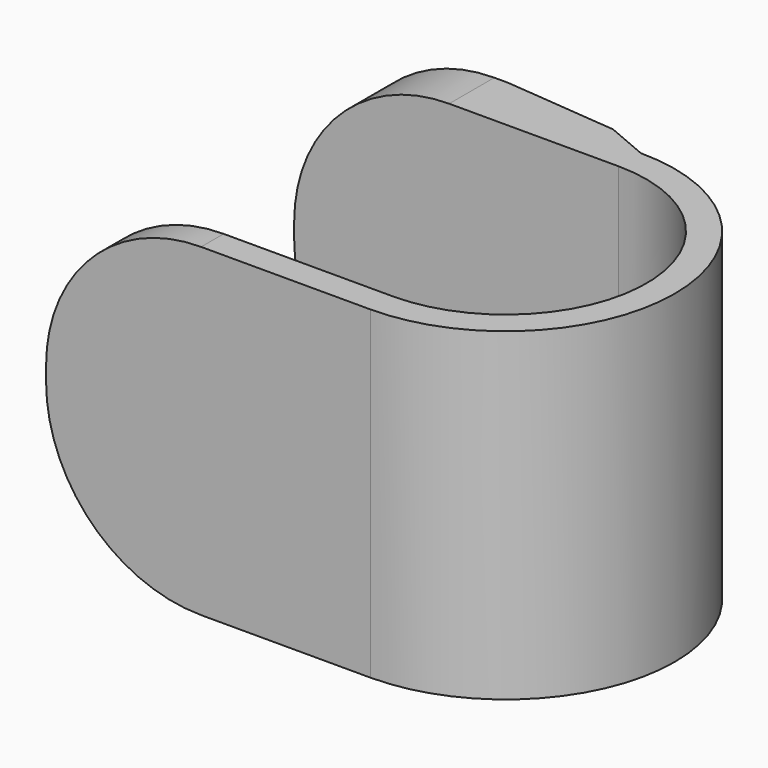
from build123d import *

# Parameters (mm, degrees)
F0_W           = 23
F0_H           = 2
F1_DEPTH       = 23
F3_D           = 1
F3_DEPTH       = 3
F3_CBORE_D     = 19.5
F3_CBORE_DEPTH = 3
F3_TIP         = 0.3004303095
F4_R           = 11
F5_T1_DEPTH    = 80.1913118923
F6_T4_DEPTH    = 38.5721694425
F6_S5_R        = 12
F6_T6_DEPTH    = 21


# Not quite as in the source:
# - a fillet or chamfer that OpenCascade refuses, or shapes differently, is made with other operations: its cross-section is extruded or revolved along the edge and cut away or added


with BuildPart() as f1:
    # F0 (on Top) → F1 (new body)
    with BuildSketch(Plane.XY):
        with BuildLine():
            Line((-8.3816226795, 2), (-8.3816226795, 0))
            Line((-8.3816226795, 0), (14.6183773205, 0))
            ThreePointArc((14.6183773205, 0), (24.6183773205, -10), (14.6183773205, -20))
            Line((14.6183773205, -20), (-8.3816226795, -20))
            Line((-8.3816226795, -20), (-8.3816226795, -22))
            Line((-8.3816226795, -22), (14.6183773205, -22))
            ThreePointArc((14.6183773205, -22), (26.6183773205, -10), (14.6183773205, 2))
            Line((14.6183773205, 2), (-8.3816226795, 2))
        make_face()
        with Locations((3.1183773205, 3)):
            Rectangle(F0_W, F0_H)
    extrude(amount=F1_DEPTH)

    # F3
    with Locations(Plane(origin=(0, 4, 0), x_dir=(-1, 0, 0), z_dir=(0, 1, 0))):
        with Locations((-3.1183773205, 11.5)):
            CounterBoreHole(F3_D / 2, F3_CBORE_D / 2, F3_CBORE_DEPTH, depth=F3_DEPTH)
            with Locations((0, 0, -(F3_DEPTH + F3_TIP / 2))):  # 118° drill point
                Cone(0, F3_D / 2, F3_TIP, mode=Mode.SUBTRACT)

    # F4
    f4_edges = [f1.edges().sort_by_distance(p)[0] for p in [
        (-8.381623, 2, 23),
        (-8.381623, 2, 0),
        (-8.381623, -21, 0),
        (-8.381623, -21, 23),
    ]]
    fillet(f4_edges, radius=F4_R)

    # F5: chamfer of 11 x 1 on 1 edges, made by hand

    # F5_s2 → F5_t1 (cut)
    with BuildSketch(Plane.XY.offset(-28.5956559462)):
        Polygon((3.6183773205, 4), (14.6183773205, 3), (14.6183773205, 4), align=None)
    extrude(amount=F5_T1_DEPTH, mode=Mode.SUBTRACT)

    # F6: chamfer of 1 x 3 on 1 edges, made by hand


with BuildPart() as f6_tool2:
    # F6_s3 → F6_t4 (new body)
    with BuildSketch(Plane.XY.offset(-7.7860847213)):
        Polygon((11.6306977011, 3.2716072381), (14.6183773205, 2), (14.6183773205, 3), align=None)
    extrude(amount=F6_T4_DEPTH)

    # F6_s5 → F6_t6 (cut, symmetric)
    with BuildSketch(Plane.XY.offset(11.5)):
        with Locations((14.6183773205, -10)):
            Circle(F6_S5_R)
    extrude(amount=F6_T6_DEPTH, both=True, mode=Mode.SUBTRACT)


with BuildPart() as f1_1:
    add(f1.part)

    # F6_t1: cut F6_tool2
    add(f6_tool2.part, mode=Mode.SUBTRACT)


solid = f1_1.part
